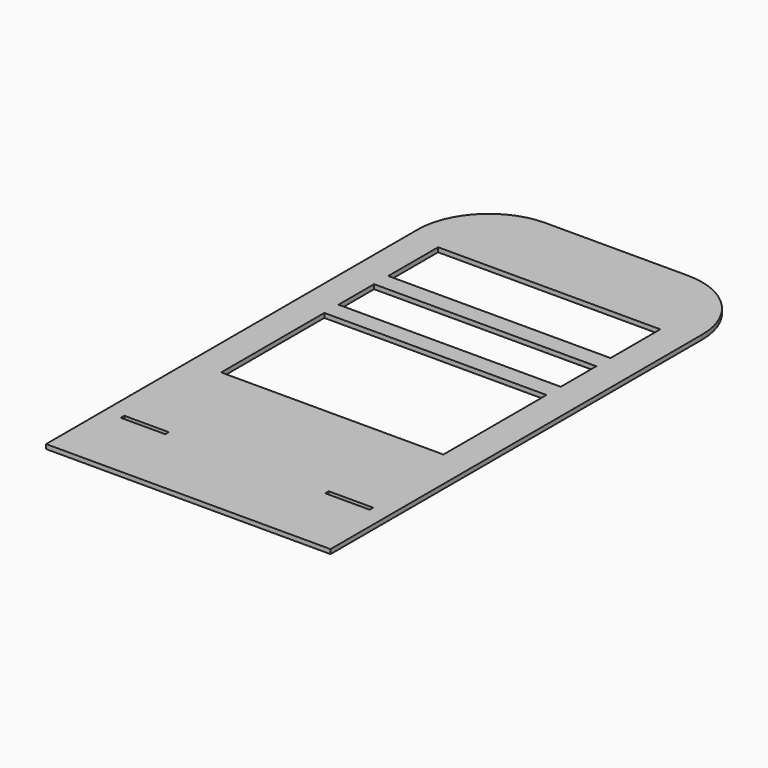
from build123d import *

# Parameters (mm, degrees)
F0_W     = 127
F0_H     = 12.7
F0_W_2   = 635
F0_H_2   = 126.9999911487
F0_H_3   = 177.8000088513
F1_DEPTH = 12.7


# Not quite as in the source:
# - a feature names something its author has since deleted; it is built from what else it names


with BuildPart() as f1:
    # F0 (on Top) → F1 (new body)
    with BuildSketch(Plane.XY):
        with BuildLine():
            ThreePointArc((-444.8386187891, 967.019580251), (-588.5227167262, 907.5036781881), (-648.0386187891, 763.819580251))
            Line((-648.0386187891, 763.819580251), (-648.0386187891, -556.980419749))
            Line((-648.0386187891, -556.980419749), (-648.0386187891, -563.330419749))
            Line((-648.0386187891, -563.330419749), (164.7613812109, -563.330419749))
            Line((164.7613812109, -563.330419749), (164.7613812109, -556.980419749))
            Line((164.7613812109, -556.980419749), (164.7613812109, 763.819580251))
            ThreePointArc((164.7613812109, 763.819580251), (105.245479148, 907.5036781881), (-38.4386187891, 967.019580251))
            Line((-38.4386187891, 967.019580251), (-444.8386187891, 967.019580251))
        make_face()
        with Locations((-533.7386187891, -353.780419749)):
            Rectangle(F0_W, F0_H, mode=Mode.SUBTRACT)
        with Locations((50.4613812109, -353.780419749)):
            Rectangle(F0_W, F0_H, mode=Mode.SUBTRACT)
        Polygon((75.8613812109, -48.980419749), (-559.1386187891, -48.980419749), (-559.1386187891, 90.719580251), (-559.1386187891, 141.519580251), (-559.1386187891, 319.319580251), (75.8613812109, 319.319580251), (75.8613812109, 141.519580251), (75.8613812109, 90.719580251), align=None, mode=Mode.SUBTRACT)
        with Locations((-241.6386187891, 433.6195758253)):
            Rectangle(F0_W_2, F0_H_2, mode=Mode.SUBTRACT)
        with Locations((-241.6386187891, 636.8195758253)):
            Rectangle(F0_W_2, F0_H_3, mode=Mode.SUBTRACT)
    extrude(amount=F1_DEPTH)


solid = f1.part
